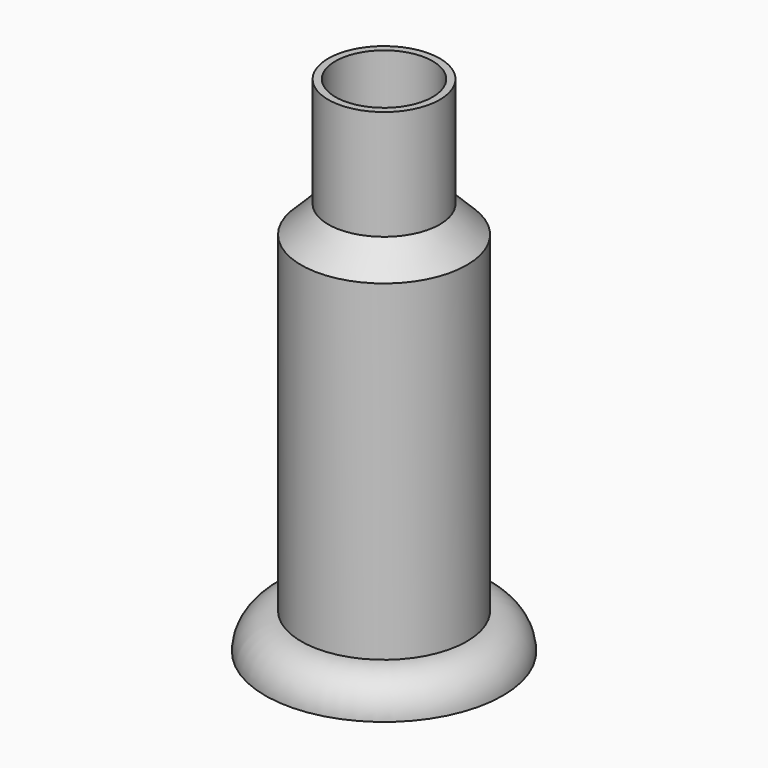
from build123d import *

# Parameters (mm, degrees)
F0_R     = 16.5
F0_R_2   = 15.5
F0_R_3   = 7.75
F1_DEPTH = 5
F2_R     = 4.99999
F3_DEPTH = 51
F0_R_4   = 6.75
F5_DEPTH = 70


# Not quite as in the source:
# - a fillet or chamfer that OpenCascade refuses, or shapes differently, is made with other operations: its cross-section is extruded or revolved along the edge and cut away or added
# - a fillet or chamfer is up to 0.001 mm smaller than in the source, because OpenCascade refuses the exact size


with BuildPart() as f1:
    # F0 (on Top) → F1 (new body)
    with BuildSketch(Plane.XY):
        Circle(F0_R)
        Circle(F0_R_2, mode=Mode.SUBTRACT)
        Circle(F0_R_2)
        Circle(F0_R_3, mode=Mode.SUBTRACT)
    extrude(amount=F1_DEPTH)

    # F2 (radius 5 in the source; OpenCascade refuses exactly that, so slightly less here)
    f2_edges = [f1.edges().sort_by_distance(p)[0] for p in [
        (-16.5, 0, 5),
    ]]
    fillet(f2_edges, radius=F2_R)


with BuildPart() as f3:
    # F3 (new): a face of the model
    f3_faces = [f1.part.faces().sort_by_distance(p)[0] for p in [
        (-11.1747405978, 0, 5),
    ]]
    extrude(f3_faces, amount=F3_DEPTH)

    # F4: chamfer of 5 on 1 edges, made by hand

    # F4_s1 → F4_t2 (revolve, cut)
    with BuildSketch(Plane.XZ):
        Polygon((11.50001, 51), (6.50001, 56), (11.50001, 56), align=None)
    revolve(axis=Axis((0, 0, 56), (0, 0, 1)), mode=Mode.SUBTRACT)


with BuildPart() as f1_1:
    add(f1.part)

    # F0 (on Top) → F5 (join)
    with BuildSketch(Plane.XY):
        Circle(F0_R_3)
        Circle(F0_R_4, mode=Mode.SUBTRACT)
    extrude(amount=F5_DEPTH)


solid = Compound([f3.part, f1_1.part])
